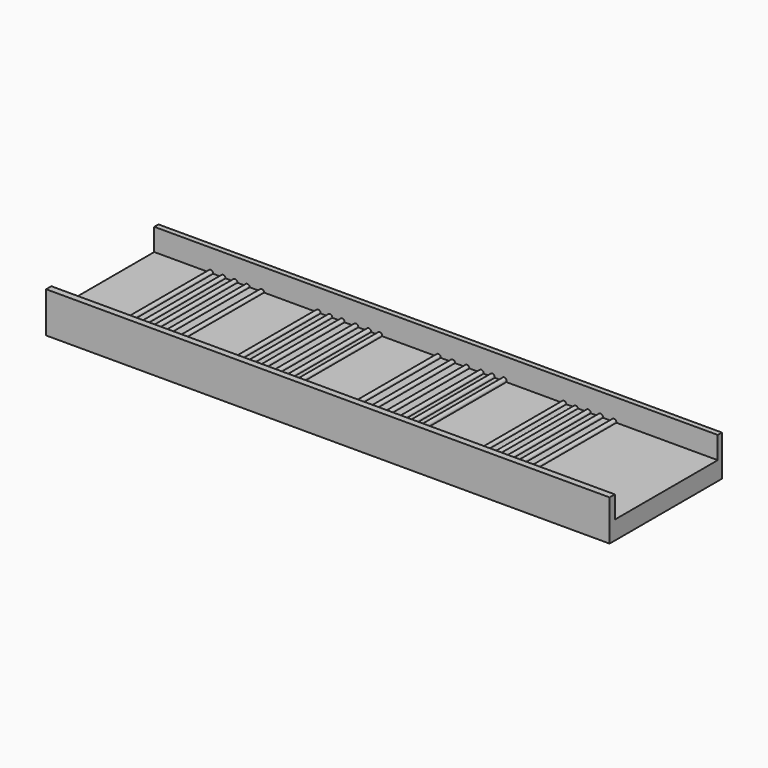
from build123d import *

# Parameters (mm, degrees)
F0_W     = 152.2748842835
F0_H     = 37.9443131387
F1_DEPTH = 5
F5_R     = 0.6498911682
F6_DEPTH = 37.9
F2_W     = 152.2748842835
F2_H     = 1.4094897779
F2_H_2   = 1.7610266805
F7_DEPTH = 6


# Not quite as in the source:
# - the program builds the solid bodies; features that only make, move or delete a surface that nothing else refers to are left out


with BuildPart() as f1:
    # F0 (on Top) → F1 (new body)
    with BuildSketch(Plane.XY):
        with Locations((0.995259732, -18.9721565694)):
            Rectangle(F0_W, F0_H)
    extrude(amount=F1_DEPTH)

    # F5 (on Front) → F6 (join)
    with BuildSketch(Plane.XZ):
        with Locations((-59.8872974515, 5.076338537)):
            Circle(F5_R)
        with Locations((-56.5108135343, 4.9978159368)):
            Circle(F5_R)
        with Locations((-46.1065284908, 4.9978159368)):
            Circle(F5_R)
        with Locations((-49.9934107065, 4.958554171)):
            Circle(F5_R)
        with Locations((-53.3306375146, 5.0370772369)):
            Circle(F5_R)
        with Locations((-30.849635601, 5.0810105167)):
            Circle(F5_R)
        with Locations((-14.1990464181, 5.1284483634)):
            Circle(F5_R)
        with Locations((-17.1876139939, 5.0810105167)):
            Circle(F5_R)
        with Locations((-20.650556311, 5.0810105167)):
            Circle(F5_R)
        with Locations((-24.3506878614, 5.0810105167)):
            Circle(F5_R)
        with Locations((-27.6713185012, 5.0335731357)):
            Circle(F5_R)
        with Locations((1.6279553529, 5.0831306726)):
            Circle(F5_R)
        with Locations((19.4284114987, 5.2831359208)):
            Circle(F5_R)
        with Locations((16.2283293903, 5.1497989334)):
            Circle(F5_R)
        with Locations((13.2282525301, 5.0831306726)):
            Circle(F5_R)
        with Locations((9.361486882, 5.0164619461)):
            Circle(F5_R)
        with Locations((5.4947216995, 5.0164619461)):
            Circle(F5_R)
        with Locations((49.0938574076, 5.0953882746)):
            Circle(F5_R)
        with Locations((45.4649962485, 5.1608970389)):
            Circle(F5_R)
        with Locations((42.1599261463, 5.0851320848)):
            Circle(F5_R)
        with Locations((38.728825748, 4.870061297)):
            Circle(F5_R)
        with Locations((35.5742499232, 4.9827247858)):
            Circle(F5_R)
    extrude(amount=F6_DEPTH)

    # F2 (on face) → F7 (join)
    with BuildSketch(Plane.XY.offset(5)):
        with Locations((0.995259732, -0.7047448889)):
            Rectangle(F2_W, F2_H)
        with Locations((0.995259732, -37.0637997985)):
            Rectangle(F2_W, F2_H_2)
    extrude(amount=F7_DEPTH)


solid = f1.part
